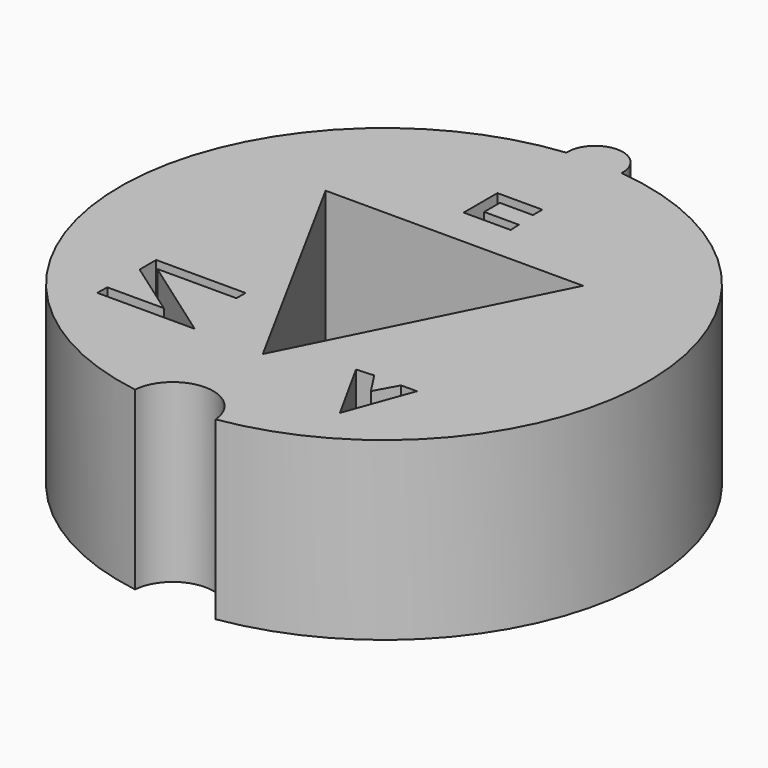
from build123d import *

# Parameters (mm, degrees)
F0_W      = 38.1
F0_H      = 25.4
F3_DEPTH  = 73.8923922181
F5_DEPTH  = 25.4
F7_DEPTH  = 25.4
F9_DEPTH  = 25.4
F11_DEPTH = 25.4
F13_DEPTH = 25.4


# Not quite as in the source:
# - ends of sketch curves that miss each other by under 0.0002 mm in the source are joined


with BuildPart() as f1:
    # F0 (on Front) → F1 (revolve)
    with BuildSketch(Plane.XZ):
        with Locations((19.05, 12.7)):
            Rectangle(F0_W, F0_H)
    revolve(axis=Axis((0, 0, 12.7), (0, 0, -1)))

    # F2 (on Top) → F3 (cut)
    with BuildSketch(Plane.XY):
        Polygon((-19.3802006543, 13.6906001717), (0, -21.8694005162), (17.7799984813, 13.6905994838), align=None)
    extrude(amount=F3_DEPTH, mode=Mode.SUBTRACT)

    # F4 (on face) → F5 (cut)
    with BuildSketch(Plane(origin=(0, 0, 0), x_dir=(1, 0, 0), z_dir=(0, 0, -1))):
        Polygon((-9.8248589784, 21.8694005162), (-23.8991640508, 21.8694005162), (-23.8595362753, 20.1035637146), (-15.7059820649, 20.1035637146), (-23.725675419, 14.439499937), (-23.725675419, 11.4520248026), (-10.8296805993, 11.4520248026), (-10.8296805993, 13.090708293), (-22.2545247525, 13.090708293), align=None)
    extrude(amount=-F5_DEPTH, mode=Mode.SUBTRACT)

    # F6 (on face) → F7 (cut)
    with BuildSketch(Plane(origin=(0, 0, 0), x_dir=(1, 0, 0), z_dir=(0, 0, -1))):
        Polygon((15.7712604851, 27.6608336717), (10.5691235512, 18.2647015899), (13.062780723, 18.0983748287), (15.1800094172, 21.327663213), (16.9541146606, 18.1070137769), (19.2498695105, 18.1070137769), align=None)
    extrude(amount=-F7_DEPTH, mode=Mode.SUBTRACT)

    # F8 (on face) → F9 (cut)
    with BuildSketch(Plane(origin=(0, 0, 0), x_dir=(1, 0, 0), z_dir=(0, 0, -1))):
        Polygon((2.8216354549, -20.8048354834), (2.9142363928, -19.2329455167), (-3.8865676615, -19.2329455167), (-3.8865676615, -25.3260713071), (2.5894464925, -25.3260713071), (2.5894464925, -23.6380007118), (-2.1816743538, -23.6380007118), (-2.1816743538, -20.8048354834), align=None)
    extrude(amount=-F9_DEPTH, mode=Mode.SUBTRACT)

    # F10 (on face) → F11 (cut)
    with BuildSketch(Plane(origin=(0, 0, 0), x_dir=(1, 0, 0), z_dir=(0, 0, -1))):
        with BuildLine():
            ThreePointArc((5.8152880434, 37.6535844904), (0, 38.1), (-5.8152880434, 37.6535844904))
            ThreePointArc((-5.8152880434, 37.6535844904), (0, 32.267602394), (5.8152880434, 37.6535844904))
        make_face()
        with BuildLine():
            ThreePointArc((5.8152880434, 37.6535844904), (5.8281186457, 37.8766283677), (5.832397606, 38.1))
            ThreePointArc((5.832397606, 38.1), (-0.2233716323, 43.9281186457), (-5.8152880434, 37.6535844904))
            ThreePointArc((-5.8152880434, 37.6535844904), (0, 38.1), (5.8152880434, 37.6535844904))
        make_face()
    extrude(amount=-F11_DEPTH, mode=Mode.SUBTRACT)

    # F12 (on face) → F13 (join)
    with BuildSketch(Plane(origin=(0, 0, 0), x_dir=(1, 0, 0), z_dir=(0, 0, -1))):
        with BuildLine():
            ThreePointArc((-3.9919458032, -37.8902938588), (0, -38.1), (3.9919458032, -37.8902938588))
            ThreePointArc((3.9919458032, -37.8902938588), (0, -34.1025498176), (-3.9919458032, -37.8902938588))
        make_face()
        with BuildLine():
            ThreePointArc((-3.9919458032, -37.8902938588), (-0.1048891842, -42.0960738507), (3.9974501824, -38.1))
            ThreePointArc((3.9974501824, -38.1), (3.9960738507, -37.9951108158), (3.9919458032, -37.8902938588))
            ThreePointArc((3.9919458032, -37.8902938588), (0, -38.1), (-3.9919458032, -37.8902938588))
        make_face()
    extrude(amount=-F13_DEPTH)


solid = f1.part
